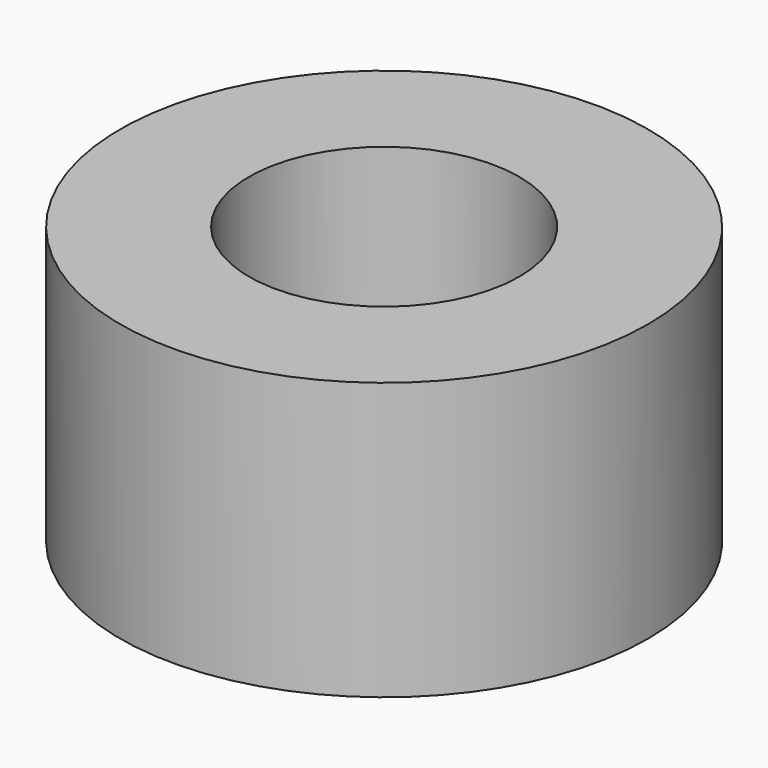
from build123d import *

# Parameters (mm, degrees)
F0_R     = 4.1
F0_R_2   = 2.1
F2_DEPTH = 4.3


# Not quite as in the source:
# - the program builds the solid bodies; features that only make, move or delete a surface that nothing else refers to are left out


with BuildPart() as f2:
    # F0 (on Top) → F2 (new body)
    with BuildSketch(Plane.XY):
        Circle(F0_R)
        Circle(F0_R_2, mode=Mode.SUBTRACT)
    extrude(amount=F2_DEPTH)


solid = f2.part
